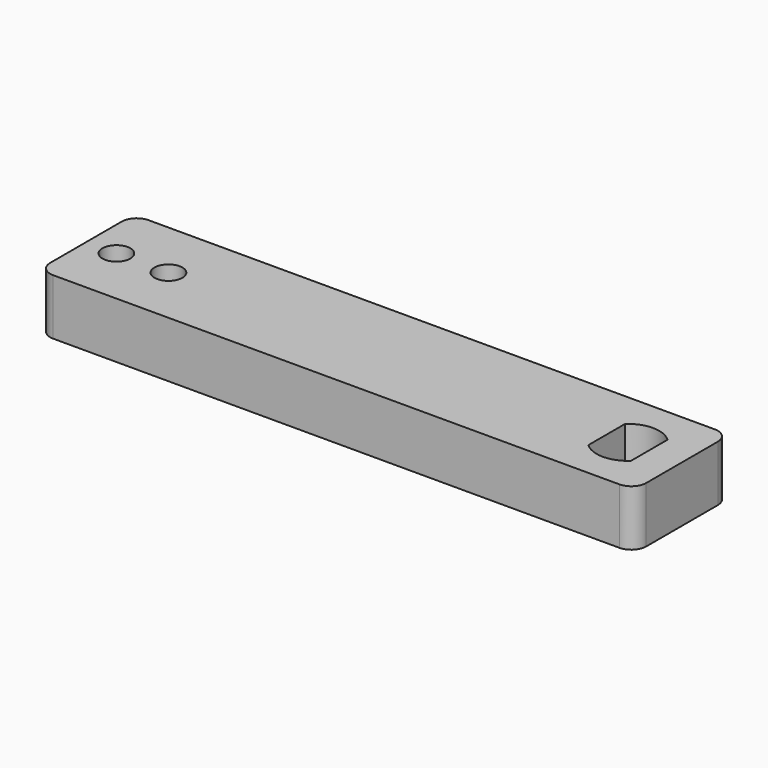
from build123d import *

# Parameters (mm, degrees)
F1_DEPTH = 4.7625
F2_R     = 1.27


# Not quite as in the source:
# - a length typed as a fraction of an inch, garbled in the dataset ("3 / 203.2 mm" for 3/8 in), is restored


with BuildPart() as f1:
    # F0 (on Top) → F1 (new body)
    with BuildSketch(Plane.XY):
        with BuildLine():
            Line((25.4, 0), (25.4, 5.08))
            Line((25.4, 5.08), (-25.4, 5.08))
            Line((-25.4, 5.08), (-25.4, 0))
            Line((-25.4, 0), (-23.9999255717, 0))
            ThreePointArc((-23.9999255717, 0), (-22.8093005717, 1.190625), (-21.6186755717, 0))
            Line((-21.6186755717, 0), (-19.5611937523, 0))
            ThreePointArc((-19.5611937523, 0), (-18.3705687523, 1.190625), (-17.1799437523, 0))
            Line((-17.1799437523, 0), (18.1277101444, 0))
            ThreePointArc((18.1277101444, 0), (18.3496715251, 1.0652113171), (18.9786101444, 1.9531179662))
            ThreePointArc((18.9786101444, 1.9531179662), (20.7947101444, 2.667), (22.6108101444, 1.9531179662))
            ThreePointArc((22.6108101444, 1.9531179662), (23.2397487637, 1.0652113171), (23.4617101444, 0))
            Line((23.4617101444, 0), (25.4, 0))
        make_face()
        with BuildLine():
            Line((18.1277101444, 0), (18.9786101444, 0))
            Line((18.9786101444, 0), (18.9786101444, 1.9531179662))
            ThreePointArc((18.9786101444, 1.9531179662), (18.3496715251, 1.0652113171), (18.1277101444, 0))
        make_face()
        with BuildLine():
            Line((18.9786101444, -1.9531179662), (18.9786101444, 0))
            Line((18.9786101444, 0), (18.1277101444, 0))
            ThreePointArc((18.1277101444, 0), (18.3496715251, -1.0652113171), (18.9786101444, -1.9531179662))
        make_face()
        with BuildLine():
            Line((22.6108101444, 0), (23.4617101444, 0))
            ThreePointArc((23.4617101444, 0), (23.2397487637, 1.0652113171), (22.6108101444, 1.9531179662))
            Line((22.6108101444, 1.9531179662), (22.6108101444, 0))
        make_face()
        with BuildLine():
            ThreePointArc((22.6108101444, -1.9531179662), (23.2397487637, -1.0652113171), (23.4617101444, 0))
            Line((23.4617101444, 0), (22.6108101444, 0))
            Line((22.6108101444, 0), (22.6108101444, -1.9531179662))
        make_face()
        with BuildLine():
            Line((25.4, -5.08), (25.4, 0))
            Line((25.4, 0), (23.4617101444, 0))
            ThreePointArc((23.4617101444, 0), (23.2397487637, -1.0652113171), (22.6108101444, -1.9531179662))
            ThreePointArc((22.6108101444, -1.9531179662), (20.7947101444, -2.667), (18.9786101444, -1.9531179662))
            ThreePointArc((18.9786101444, -1.9531179662), (18.3496715251, -1.0652113171), (18.1277101444, 0))
            Line((18.1277101444, 0), (-17.1799437523, 0))
            ThreePointArc((-17.1799437523, 0), (-18.3705687523, -1.190625), (-19.5611937523, 0))
            Line((-19.5611937523, 0), (-21.6186755717, 0))
            ThreePointArc((-21.6186755717, 0), (-22.8093005717, -1.190625), (-23.9999255717, 0))
            Line((-23.9999255717, 0), (-25.4, 0))
            Line((-25.4, 0), (-25.4, -5.08))
            Line((-25.4, -5.08), (25.4, -5.08))
        make_face()
    extrude(amount=F1_DEPTH)

    # F2
    f2_edges = [f1.edges().sort_by_distance(p)[0] for p in [
        (25.4, 5.08, 2.38125),
        (25.4, -5.08, 2.38125),
        (-25.4, 5.08, 2.38125),
        (-25.4, -5.08, 2.38125),
    ]]
    fillet(f2_edges, radius=F2_R)


solid = f1.part
